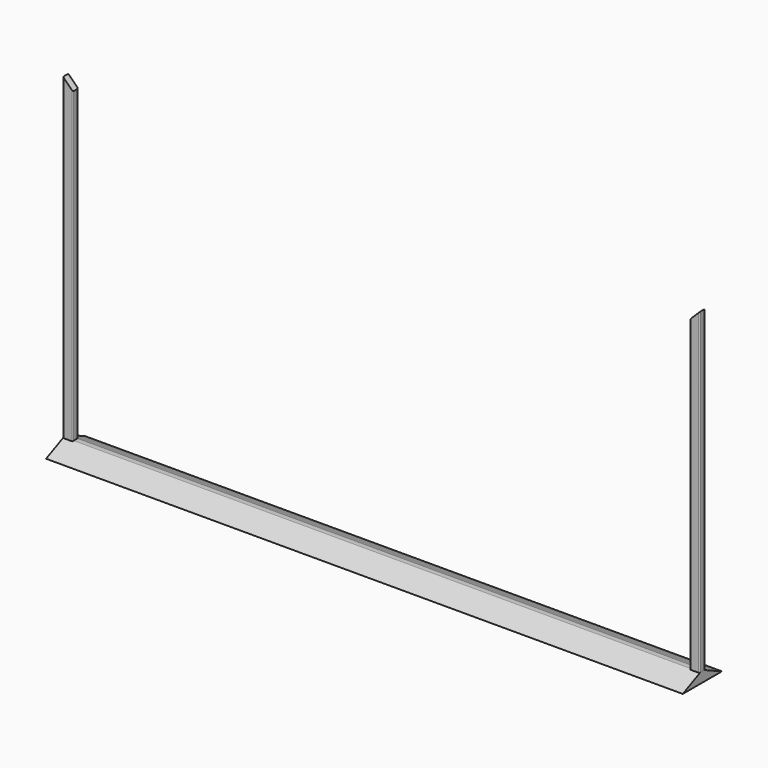
from build123d import *

# Parameters (mm, degrees)
F1_DEPTH      = 20
F3_DEPTH      = 477.5
F4_R          = 6
F4_2_R        = 6
F7_DEPTH      = 1935
F7_DEPTH_BACK = 1935
F8_W          = 3750.3852844238
F8_H          = 4.1501820087
F9_DEPTH      = 10


# Not quite as in the source:
# - a feature names something its author has since deleted; it is built from what else it names


with BuildPart() as f1:
    # F0 (on Front) → F1 (new body, symmetric)
    with BuildSketch(Plane.XZ):
        Polygon((-1875, -936), (-1875, 936), (-1935, 996), (-1935, -996), align=None)
    extrude(amount=F1_DEPTH, both=True)

    # F4
    f4_edges = [f1.edges().sort_by_distance(p)[0] for p in [
        (-1875, -20, 0),
        (-1935, -20, 0),
        (-1875, 20, 0),
        (-1935, 20, 0),
    ]]
    fillet(f4_edges, radius=F4_R)


with BuildPart() as f1b:
    # F0 (on Front) → F1, piece 2 (new body, symmetric)
    with BuildSketch(Plane.XZ):
        Polygon((1935, -996), (1935, 996), (1875, 936), (1875, -936), align=None)
    extrude(amount=F1_DEPTH, both=True)

    # F4#2
    f4_2_edges = [f1b.edges().sort_by_distance(p)[0] for p in [
        (1935, -20, 0),
        (1875, -20, 0),
        (1935, 20, 0),
        (1875, 20, 0),
    ]]
    fillet(f4_2_edges, radius=F4_2_R)


with BuildPart() as f3:
    # F2 (on Top) → F3 (new body, symmetric)
    with BuildSketch(Plane.XY):
        with BuildLine():
            ThreePointArc((-758, 14), (-758.8786796564, 16.1213203436), (-761, 17))
            Line((-761, 17), (-809, 17))
            ThreePointArc((-809, 17), (-811.1213203436, 16.1213203436), (-812, 14))
            Line((-812, 14), (-812, -14))
            ThreePointArc((-812, -14), (-811.1213203436, -16.1213203436), (-809, -17))
            Line((-809, -17), (-761, -17))
            ThreePointArc((-761, -17), (-758.8786796564, -16.1213203436), (-758, -14))
            Line((-758, -14), (-758, 14))
        make_face()
    extrude(amount=F3_DEPTH, both=True)


with BuildPart() as f3b:
    # F2 (on Top) → F3, piece 2 (new body, symmetric)
    with BuildSketch(Plane.XY):
        with BuildLine():
            ThreePointArc((809, -17), (811.1213203436, -16.1213203436), (812, -14))
            Line((812, -14), (812, 14))
            ThreePointArc((812, 14), (811.1213203436, 16.1213203436), (809, 17))
            Line((809, 17), (761, 17))
            ThreePointArc((761, 17), (758.8786796564, 16.1213203436), (758, 14))
            Line((758, 14), (758, -14))
            ThreePointArc((758, -14), (758.8786796564, -16.1213203436), (761, -17))
            Line((761, -17), (809, -17))
        make_face()
    extrude(amount=F3_DEPTH, both=True)


with BuildPart() as f1b_1:
    add(f1b.part)

    # F5: cut F3, F3b
    add(f3.part, mode=Mode.SUBTRACT)
    add(f3b.part, mode=Mode.SUBTRACT)


with BuildPart() as f1_1:
    add(f1.part)

    # F5: cut F3, F3b
    add(f3.part, mode=Mode.SUBTRACT)
    add(f3b.part, mode=Mode.SUBTRACT)

    # F8 (on face) → F9 (cut)
    with BuildSketch(Plane(origin=(0, 351.2576934301, -767.0319016123), x_dir=(1, 0, 0), z_dir=(0, -0.4163621946, 0.9091988357))):
        with Locations((-0.204205513, -176.041290164)):
            Rectangle(F8_W, F8_H)
        with Locations((-0.204205513, -171.8911081553)):
            Rectangle(F8_W, F8_H)
    extrude(amount=-F9_DEPTH, mode=Mode.SUBTRACT)


with BuildPart() as f7:
    # F6 (on Right) → F7 (new body, two sides)
    with BuildSketch(Plane.YZ) as f7_sk:
        Polygon((14.1061842442, -934.3481144905), (0, -934.3481144905), (-14.1061842442, -934.3481144905), (-148.7337350845, -996), (0, -996), (148.7337350845, -996), align=None)
    extrude(amount=F7_DEPTH)
    extrude(f7_sk.sketch, amount=-F7_DEPTH_BACK)


solid = Compound([f1b_1.part, f1_1.part, f7.part])
